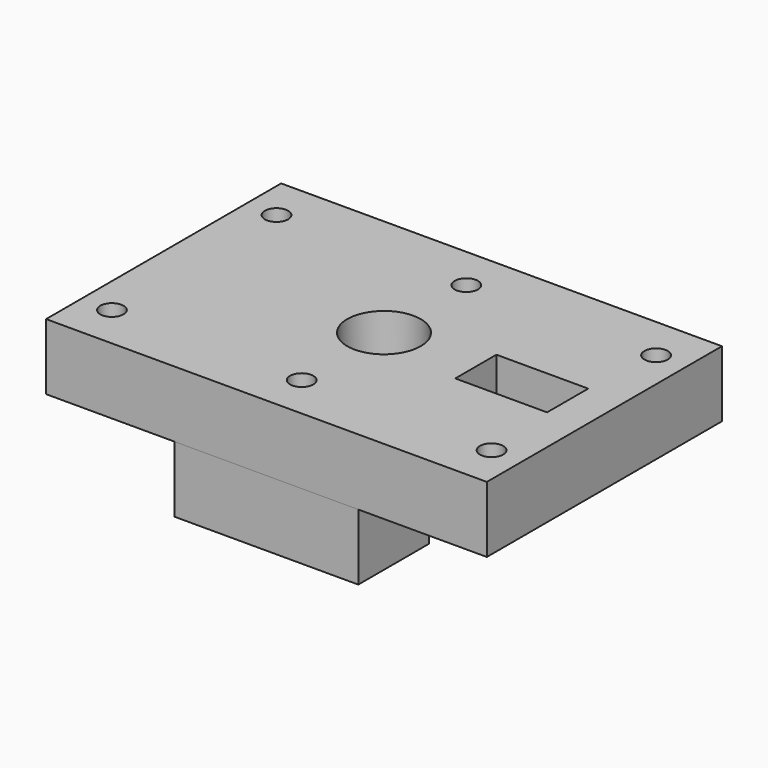
from build123d import *

# Parameters (mm, degrees)
F0_R     = 1.5875
F0_R_2   = 8
F0_W     = 12.5
F0_H     = 7
F1_DEPTH = 9
F0_R_3   = 5
F2_DEPTH = 5.2
F3_R     = 1.5875
F4_DEPTH = 9
F5_DEPTH = 6


with BuildPart() as f1:
    # F0 (on Top) → F1 (new body)
    with BuildSketch(Plane.XY):
        Polygon((30, -20), (30, 20), (-30, 20), (-30, -20), (-24.25, -20), (24.25, -20), align=None)
        with Locations((-25.8375, -14)):
            Circle(F0_R, mode=Mode.SUBTRACT)
        with Locations((-25.8375, 14)):
            Circle(F0_R, mode=Mode.SUBTRACT)
        with Locations((0, -14)):
            Circle(F0_R, mode=Mode.SUBTRACT)
        with Locations((25.8375, -14)):
            Circle(F0_R, mode=Mode.SUBTRACT)
        Circle(F0_R_2, mode=Mode.SUBTRACT)
        with Locations((0, 14)):
            Circle(F0_R, mode=Mode.SUBTRACT)
        with Locations((18.75, 0)):
            Rectangle(F0_W, F0_H, mode=Mode.SUBTRACT)
        with Locations((25.8375, 14)):
            Circle(F0_R, mode=Mode.SUBTRACT)
    extrude(amount=-F1_DEPTH)

    # F0 (on Top) → F2 (join, through all)
    with BuildSketch(Plane.XY):
        Circle(F0_R_2)
        Circle(F0_R_3, mode=Mode.SUBTRACT)
    extrude(amount=-F2_DEPTH)


with BuildPart() as f4:
    # F3 (on face) → F4 (new body)
    with BuildSketch(Plane(origin=(0, 0, -9), x_dir=(1, 0, 0), z_dir=(0, 0, -1))):
        with BuildLine():
            Line((12.5, 20), (-12.5, 20))
            Line((-12.5, 20), (-12.5, -20))
            Line((-12.5, -20), (12.5, -20))
            Line((12.5, -20), (12.5, -8))
            Line((12.5, -8), (0, -8))
            ThreePointArc((0, -8), (-8, 0), (0, 8))
            Line((0, 8), (12.5, 8))
            Line((12.5, 8), (12.5, 20))
        make_face()
        with Locations((0, -14)):
            Circle(F3_R, mode=Mode.SUBTRACT)
        with Locations((0, 14)):
            Circle(F3_R, mode=Mode.SUBTRACT)
    extrude(amount=F4_DEPTH)

    # F3 (on face) → F5 (join)
    with BuildSketch(Plane(origin=(0, 0, -9), x_dir=(1, 0, 0), z_dir=(0, 0, -1))):
        with BuildLine():
            Line((0, -8), (12.5, -8))
            Line((12.5, -8), (12.5, -6))
            Line((12.5, -6), (5.2915026221, -6))
            ThreePointArc((5.2915026221, -6), (2.8284271247, -7.4833147735), (0, -8))
        make_face()
        with BuildLine():
            ThreePointArc((5.2915026221, 6), (2.8284271247, 7.4833147735), (0, 8))
            ThreePointArc((0, 8), (-8, 0), (0, -8))
            ThreePointArc((0, -8), (2.8284271247, -7.4833147735), (5.2915026221, -6))
            Line((5.2915026221, -6), (0, -6))
            ThreePointArc((0, -6), (-6, 0), (0, 6))
            Line((0, 6), (5.2915026221, 6))
        make_face()
        with BuildLine():
            Line((12.5, 6), (12.5, 8))
            Line((12.5, 8), (0, 8))
            ThreePointArc((0, 8), (2.8284271247, 7.4833147735), (5.2915026221, 6))
            Line((5.2915026221, 6), (12.5, 6))
        make_face()
    extrude(amount=F5_DEPTH)


solid = Compound([f1.part, f4.part])
